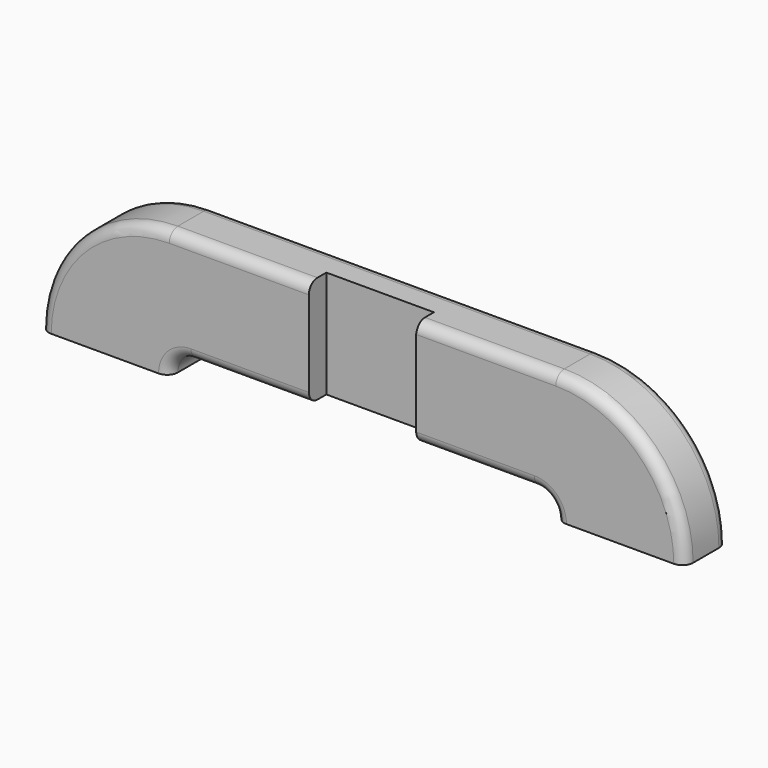
from build123d import *

# Parameters (mm, degrees)
F0_W         = 90
F0_H         = 50
F1_DEPTH     = 25
F2_R         = 59.99999
F3_R         = 9.99999
F4_R         = 9.99999
F5_R         = 59.99999
F6_T1_DEPTH  = 12.50001
F6_T3_DEPTH  = 180.00002
F6_T6_ANGLE  = 90
F6_T8_ANGLE  = 90
F7_T1_DEPTH  = 12.50001
F7_T3_DEPTH  = 180.00002
F7_T6_ANGLE  = 90
F7_T8_ANGLE  = 90
F8_T1_DEPTH  = 160.00002
F8_T3_DEPTH  = 12.50001
F8_T6_ANGLE  = 90
F8_T8_ANGLE  = 90
F8_T10_ANGLE = 90
F8_T12_ANGLE = 90
F9_W         = 50
F9_H         = 5
F9_H_2       = 40
F10_DEPTH    = 10
F13_W        = 50
F13_H        = 10
F14_DEPTH    = 60.001
F16_DEPTH    = 10


# Not quite as in the source:
# - a fillet or chamfer that OpenCascade refuses, or shapes differently, is made with other operations: its cross-section is extruded or revolved along the edge and cut away or added
# - a fillet or chamfer is up to 0.001 mm smaller than in the source, because OpenCascade refuses the exact size


with BuildPart() as f1:
    # F0 (on Front) → F1 (new body)
    with BuildSketch(Plane.XZ):
        with Locations((45, 0)):
            Rectangle(F0_W, F0_H)
        Polygon((150, 25), (90, 25), (90, -25), (90, -35), (150, -35), align=None)
        with Locations((-45, 0)):
            Rectangle(F0_W, F0_H)
        Polygon((-90, -25), (-90, 25), (-150, 25), (-150, -35), (-90, -35), align=None)
    extrude(amount=F1_DEPTH)

    # F2 (radius 60 in the source; OpenCascade refuses exactly that, so slightly less here)
    f2_edges = [f1.edges().sort_by_distance(p)[0] for p in [
        (-150, -12.5, 25),
    ]]
    fillet(f2_edges, radius=F2_R)

    # F3 (radius 10 in the source; OpenCascade refuses exactly that, so slightly less here)
    f3_edges = [f1.edges().sort_by_distance(p)[0] for p in [
        (-90, -12.5, -25),
    ]]
    fillet(f3_edges, radius=F3_R)

    # F4 (radius 10 in the source; OpenCascade refuses exactly that, so slightly less here)
    f4_edges = [f1.edges().sort_by_distance(p)[0] for p in [
        (90, -12.5, -25),
    ]]
    fillet(f4_edges, radius=F4_R)

    # F5 (radius 60 in the source; OpenCascade refuses exactly that, so slightly less here)
    f5_edges = [f1.edges().sort_by_distance(p)[0] for p in [
        (150, -12.5, 25),
    ]]
    fillet(f5_edges, radius=F5_R)

    # F6: fillet of radius 5 on 1 edges, made by hand

    # F6_s2 → F6_t1 (cut)
    with BuildSketch(Plane.XY.offset(-47.5)):
        with BuildLine():
            ThreePointArc((150, -20), (148.5355339059, -23.5355339059), (145, -25))
            Line((145, -25), (150, -25))
            Line((150, -25), (150, -20))
        make_face()
        with BuildLine():
            ThreePointArc((-150, -20), (-148.5355339059, -23.5355339059), (-145, -25))
            Line((-145, -25), (-150, -25))
            Line((-150, -25), (-150, -20))
        make_face()
    extrude(amount=F6_T1_DEPTH, mode=Mode.SUBTRACT)

    # F6_s4 → F6_t3 (cut)
    with BuildSketch(Plane.YZ.offset(-90.00001)):
        with BuildLine():
            ThreePointArc((-20, 25), (-23.5355339059, 23.5355339059), (-25, 20))
            Line((-25, 20), (-25, 25))
            Line((-25, 25), (-20, 25))
        make_face()
    extrude(amount=F6_T3_DEPTH, mode=Mode.SUBTRACT)

    # F6_s5 → F6_t6 (revolve, cut)
    with BuildSketch(Plane.XY.offset(-34.99999)):
        with BuildLine():
            ThreePointArc((150, -20), (148.5355339059, -23.5355339059), (145, -25))
            Line((145, -25), (150, -25))
            Line((150, -25), (150, -20))
        make_face()
    revolve(axis=Axis((90.00001, -25, -34.99999), (0, -1, 0)), revolution_arc=F6_T6_ANGLE, mode=Mode.SUBTRACT)

    # F6_s7 → F6_t8 (revolve, cut)
    with BuildSketch(Plane.YZ.offset(-90.00001)):
        with BuildLine():
            ThreePointArc((-20, 25), (-23.5355339059, 23.5355339059), (-25, 20))
            Line((-25, 20), (-25, 25))
            Line((-25, 25), (-20, 25))
        make_face()
    revolve(axis=Axis((-90.00001, -25, -34.99999), (0, -1, 0)), revolution_arc=F6_T8_ANGLE, mode=Mode.SUBTRACT)

    # F7: fillet of radius 5 on 1 edges, made by hand

    # F7_s2 → F7_t1 (cut)
    with BuildSketch(Plane.XY.offset(-47.5)):
        with BuildLine():
            ThreePointArc((145, 0), (148.5355339059, -1.4644660941), (150, -5))
            Line((150, -5), (150, 0))
            Line((150, 0), (145, 0))
        make_face()
        with BuildLine():
            ThreePointArc((-145, 0), (-148.5355339059, -1.4644660941), (-150, -5))
            Line((-150, -5), (-150, 0))
            Line((-150, 0), (-145, 0))
        make_face()
    extrude(amount=F7_T1_DEPTH, mode=Mode.SUBTRACT)

    # F7_s4 → F7_t3 (cut)
    with BuildSketch(Plane.YZ.offset(-90.00001)):
        with BuildLine():
            ThreePointArc((0, 20), (-1.4644660941, 23.5355339059), (-5, 25))
            Line((-5, 25), (0, 25))
            Line((0, 25), (0, 20))
        make_face()
    extrude(amount=F7_T3_DEPTH, mode=Mode.SUBTRACT)

    # F7_s5 → F7_t6 (revolve, cut)
    with BuildSketch(Plane.XY.offset(-34.99999)):
        with BuildLine():
            ThreePointArc((145, 0), (148.5355339059, -1.4644660941), (150, -5))
            Line((150, -5), (150, 0))
            Line((150, 0), (145, 0))
        make_face()
    revolve(axis=Axis((90.00001, 0, -34.99999), (0, -1, 0)), revolution_arc=F7_T6_ANGLE, mode=Mode.SUBTRACT)

    # F7_s7 → F7_t8 (revolve, cut)
    with BuildSketch(Plane.YZ.offset(-90.00001)):
        with BuildLine():
            ThreePointArc((0, 20), (-1.4644660941, 23.5355339059), (-5, 25))
            Line((-5, 25), (0, 25))
            Line((0, 25), (0, 20))
        make_face()
    revolve(axis=Axis((-90.00001, 0, -34.99999), (0, -1, 0)), revolution_arc=F7_T8_ANGLE, mode=Mode.SUBTRACT)

    # F8: fillet of radius 5 on 2 edges, made by hand

    # F8_s2 → F8_t1 (cut)
    with BuildSketch(Plane.YZ.offset(-80.00001)):
        with BuildLine():
            ThreePointArc((-20, -25), (-23.5355339059, -23.5355339059), (-25, -20))
            Line((-25, -20), (-25, -25))
            Line((-25, -25), (-20, -25))
        make_face()
        with BuildLine():
            ThreePointArc((0, -20), (-1.4644660941, -23.5355339059), (-5, -25))
            Line((-5, -25), (0, -25))
            Line((0, -25), (0, -20))
        make_face()
    extrude(amount=F8_T1_DEPTH, mode=Mode.SUBTRACT)

    # F8_s4 → F8_t3 (cut)
    with BuildSketch(Plane.XY.offset(-47.5)):
        with BuildLine():
            ThreePointArc((90, -20), (91.4644660941, -23.5355339059), (95, -25))
            Line((95, -25), (90, -25))
            Line((90, -25), (90, -20))
        make_face()
        with BuildLine():
            ThreePointArc((-90, -20), (-91.4644660941, -23.5355339059), (-95, -25))
            Line((-95, -25), (-90, -25))
            Line((-90, -25), (-90, -20))
        make_face()
        with BuildLine():
            ThreePointArc((95, 0), (91.4644660941, -1.4644660941), (90, -5))
            Line((90, -5), (90, 0))
            Line((90, 0), (95, 0))
        make_face()
        with BuildLine():
            ThreePointArc((-95, 0), (-91.4644660941, -1.4644660941), (-90, -5))
            Line((-90, -5), (-90, 0))
            Line((-90, 0), (-95, 0))
        make_face()
    extrude(amount=F8_T3_DEPTH, mode=Mode.SUBTRACT)

    # F8_s5 → F8_t6 (revolve, cut)
    with BuildSketch(Plane.YZ.offset(80.00001)):
        with BuildLine():
            ThreePointArc((0, -20), (-1.4644660941, -23.5355339059), (-5, -25))
            Line((-5, -25), (0, -25))
            Line((0, -25), (0, -20))
        make_face()
    revolve(axis=Axis((80.00001, 0, -34.99999), (0, 1, 0)), revolution_arc=F8_T6_ANGLE, mode=Mode.SUBTRACT)

    # F8_s7 → F8_t8 (revolve, cut)
    with BuildSketch(Plane.XY.offset(-34.99999)):
        with BuildLine():
            ThreePointArc((-90, -20), (-91.4644660941, -23.5355339059), (-95, -25))
            Line((-95, -25), (-90, -25))
            Line((-90, -25), (-90, -20))
        make_face()
    revolve(axis=Axis((-80.00001, -25, -34.99999), (0, 1, 0)), revolution_arc=F8_T8_ANGLE, mode=Mode.SUBTRACT)

    # F8_s9 → F8_t10 (revolve, cut)
    with BuildSketch(Plane.YZ.offset(80.00001)):
        with BuildLine():
            ThreePointArc((-20, -25), (-23.5355339059, -23.5355339059), (-25, -20))
            Line((-25, -20), (-25, -25))
            Line((-25, -25), (-20, -25))
        make_face()
    revolve(axis=Axis((80.00001, -25, -34.99999), (0, 1, 0)), revolution_arc=F8_T10_ANGLE, mode=Mode.SUBTRACT)

    # F8_s11 → F8_t12 (revolve, cut)
    with BuildSketch(Plane.XY.offset(-34.99999)):
        with BuildLine():
            ThreePointArc((-95, 0), (-91.4644660941, -1.4644660941), (-90, -5))
            Line((-90, -5), (-90, 0))
            Line((-90, 0), (-95, 0))
        make_face()
    revolve(axis=Axis((-80.00001, 0, -34.99999), (0, 1, 0)), revolution_arc=F8_T12_ANGLE, mode=Mode.SUBTRACT)

    # F9 (on face) → F10 (join)
    with BuildSketch(Plane.XZ.offset(25)):
        with Locations((0, -22.5)):
            Rectangle(F9_W, F9_H)
        with Locations((0, 22.5)):
            Rectangle(F9_W, F9_H)
        Rectangle(F9_W, F9_H_2)
    extrude(amount=-F10_DEPTH)

    # F13 (on face) → F14 (cut, through all)
    with BuildSketch(Plane.XY.offset(25)):
        with Locations((0.0907536596, -19.8229007973)):
            Rectangle(F13_W, F13_H)
    extrude(amount=-F14_DEPTH, mode=Mode.SUBTRACT)

    # F15 (on face) → F16 (cut)
    with BuildSketch(Plane.XZ.offset(25)):
        Polygon((25, 25), (-25, 25), (-25, 20), (-25, -20), (-25, -25), (25, -25), (25, -20), (25, 20), align=None)
    extrude(amount=-F16_DEPTH, mode=Mode.SUBTRACT)


solid = f1.part
